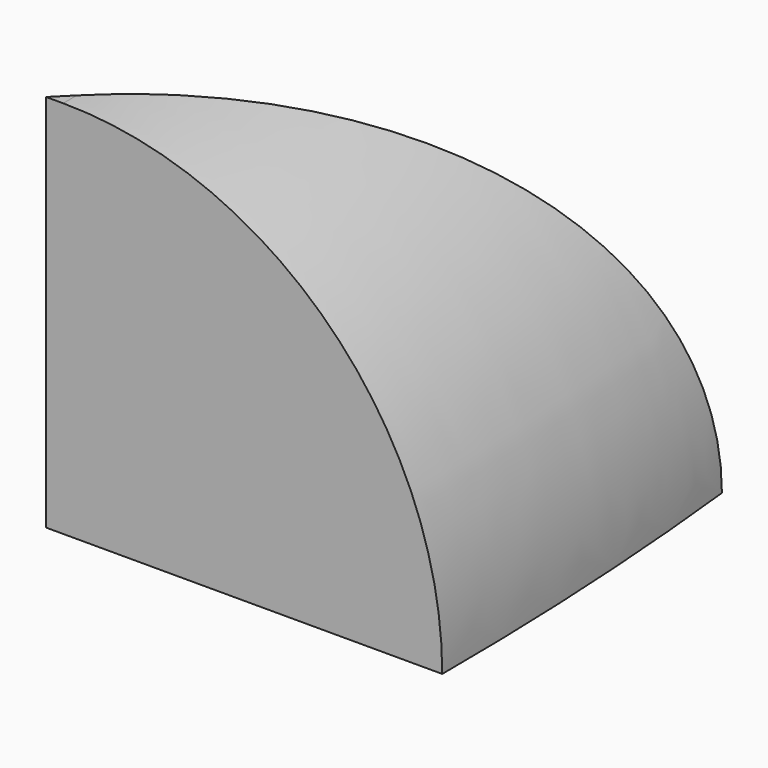
from build123d import *

# Parameters (mm, degrees)
F2_DEPTH = 25.4
F3_R     = 25.39999


# Not quite as in the source:
# - a fillet or chamfer is up to 0.001 mm smaller than in the source, because OpenCascade refuses the exact size


with BuildPart() as f2:
    # F1 (on face) → F2 (new body)
    with BuildSketch(Plane.XY):
        with BuildLine():
            Line((202.0557627241, 0), (228.6, 0))
            ThreePointArc((228.6, 0), (228.2526522951, 12.5970917379), (227.2116647397, 25.1559020156))
            Line((227.2116647397, 25.1559020156), (202.0557627241, 0))
        make_face()
    extrude(amount=F2_DEPTH)

    # F3 (radius 25.4 in the source; OpenCascade refuses exactly that, so slightly less here)
    f3_edges = [f2.edges().sort_by_distance(p)[0] for p in [
        (228.252652, 12.597092, 25.4),
    ]]
    fillet(f3_edges, radius=F3_R)


solid = f2.part
